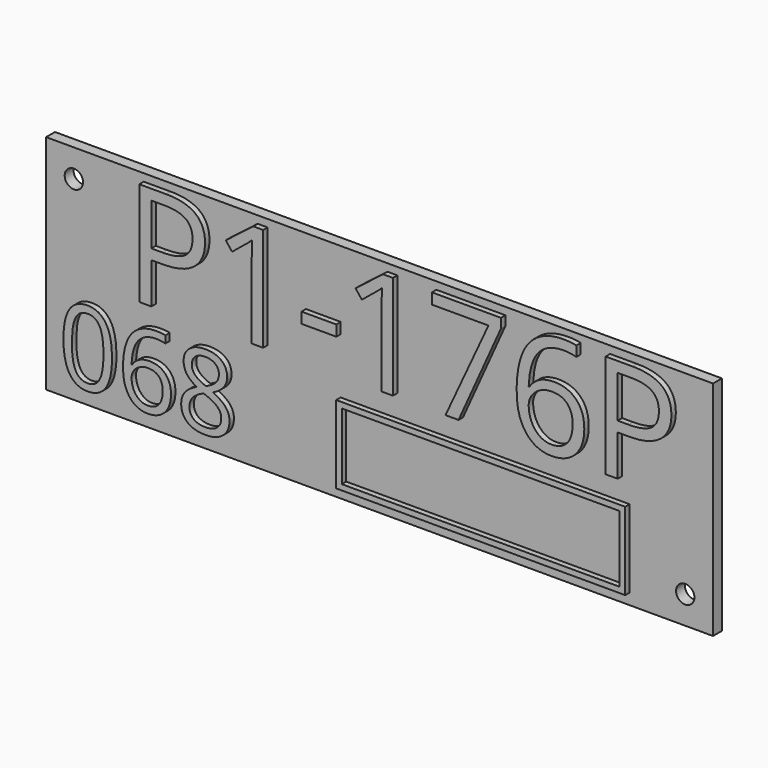
from build123d import *

# Parameters (mm, degrees)
F0_W         = 120
F0_H         = 40
F1_DEPTH     = 2
F3_D         = 3.3
F4_TEXT_SIZE = 26.1352499183
F5_DEPTH     = 1
F6_TEXT_SIZE = 18.5155049272
F7_DEPTH     = 1
F8_W         = 52
F8_H         = 14
F8_W_2       = 49.99999962
F8_H_2       = 11.99999962
F9_DEPTH     = 1


# Not quite as in the source:
# - Text() gives the source's letters only with a copy of the font that has no kerning and outlines rounded to 1/6400 em; it was checked with that copy


with BuildPart() as f1:
    # F0 (on Front) → F1 (new body)
    with BuildSketch(Plane.XZ):
        Rectangle(F0_W, F0_H)
    extrude(amount=F1_DEPTH)

    # F3 (through all)
    with Locations(Plane.XZ.offset(2)):
        with Locations((-55, 15), (55, -15)):
            Hole(F3_D / 2)

    # F4 (on face) → F5 (join)
    with BuildSketch(Plane.XZ.offset(2)):
        with Locations((-45, 0)):
            Text('P1-176P', F4_TEXT_SIZE, font='Open Sans', text_align=(TextAlign.LEFT, TextAlign.BOTTOM))
    extrude(amount=F5_DEPTH)

    # F6 (on face) → F7 (join)
    with BuildSketch(Plane.XZ.offset(2)):
        with Locations((-57, -17)):
            Text('068', F6_TEXT_SIZE, font='Open Sans', text_align=(TextAlign.LEFT, TextAlign.BOTTOM))
    extrude(amount=F7_DEPTH)

    # F8 (on face) → F9 (join)
    with BuildSketch(Plane.XZ.offset(2)):
        with Locations((19, -11)):
            Rectangle(F8_W, F8_H)
        with Locations((19, -11)):
            Rectangle(F8_W_2, F8_H_2, mode=Mode.SUBTRACT)
    extrude(amount=F9_DEPTH)


solid = f1.part
